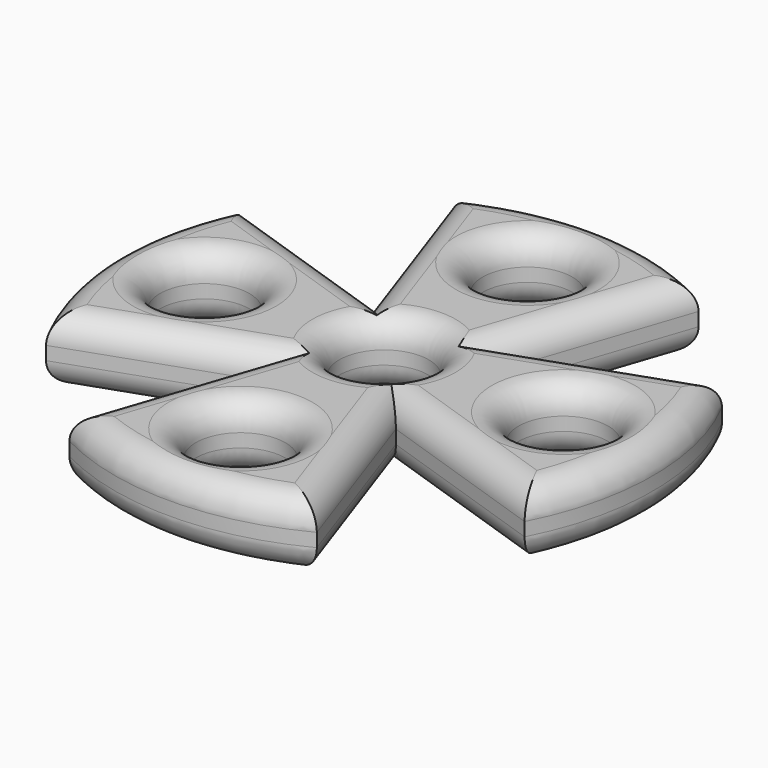
from build123d import *

# Parameters (mm, degrees)
F0_R          = 38.1
F1_DEPTH      = 9.525
F2_R          = 6.35
F3_DEPTH      = 25.4
F4_R          = 6.35
F5_DEPTH      = 25.4
F6_T2_ANGLE   = 83.3157190196
F6_T6_DEPTH   = 45.2852726424
F6_T11_DEPTH  = 45.38242659
F6_T14_ANGLE  = 83.3157190196
F6_T18_DEPTH  = 45.2852726424
F6_T23_DEPTH  = 45.38242659
F6_T26_ANGLE  = 83.3157190196
F6_T30_DEPTH  = 45.2852726424
F6_T35_DEPTH  = 45.38242659
F6_T38_ANGLE  = 83.3157190196
F6_T42_DEPTH  = 45.2852726424
F6_T47_DEPTH  = 45.38242659
F6_T62_DEPTH  = 45.38242659
F6_T65_ANGLE  = 83.3157190196
F6_T69_DEPTH  = 45.2852726424
F6_T74_DEPTH  = 45.38242659
F6_T77_ANGLE  = 83.3157190196
F6_T81_DEPTH  = 45.2852726424
F6_T86_DEPTH  = 45.38242659
F6_T89_ANGLE  = 83.3157190196
F6_T93_DEPTH  = 45.2852726424
F6_T98_DEPTH  = 45.38242659
F6_T101_ANGLE = 83.3157190196
F6_T105_DEPTH = 45.2852726424
F6_T121_DEPTH = 45.2852726424
F6_T125_DEPTH = 45.38242659
F6_T132_DEPTH = 45.2852726424
F6_T136_DEPTH = 45.38242659
F6_T143_DEPTH = 45.2852726424
F6_T147_DEPTH = 45.38242659
F6_T154_DEPTH = 45.2852726424
F6_T158_DEPTH = 45.38242659
F6_T165_DEPTH = 45.2852726424
F6_T169_DEPTH = 45.38242659
F6_T176_DEPTH = 45.2852726424
F6_T180_DEPTH = 45.38242659
F6_T187_DEPTH = 45.2852726424
F6_T191_DEPTH = 45.38242659
F6_T198_DEPTH = 45.2852726424
F6_T202_DEPTH = 45.38242659


# Not quite as in the source:
# - a fillet or chamfer that OpenCascade refuses, or shapes differently, is made with other operations: its cross-section is extruded or revolved along the edge and cut away or added


with BuildPart() as f1:
    # F0 (on Top) → F1 (new body)
    with BuildSketch(Plane.XY):
        Circle(F0_R)
    extrude(amount=F1_DEPTH)

    # F2 (on Top) → F3 (cut)
    with BuildSketch(Plane.XY):
        Circle(F2_R)
    extrude(amount=F3_DEPTH, mode=Mode.SUBTRACT)

    # F4 (on Top) → F5 (cut)
    with BuildSketch(Plane.XY):
        with Locations((-25.4, 0)):
            Circle(F4_R)
        with Locations((0, -25.4)):
            Circle(F4_R)
        with Locations((25.4, 0)):
            Circle(F4_R)
        with Locations((0, 25.4)):
            Circle(F4_R)
        Polygon((-17.7651587874, 34.4617366791), (-44.7468273342, 21.1044754833), (-8.9149055738, 9.045134527), align=None)
        Polygon((-34.4617366791, -17.7651587874), (-21.1044754833, -44.7468273342), (-9.045134527, -8.9149055738), align=None)
        Polygon((17.7651587874, -34.4617366791), (44.7468273342, -21.1044754833), (8.9149055738, -9.045134527), align=None)
        Polygon((34.4617366791, 17.7651587874), (21.1044754833, 44.7468273342), (9.045134527, 8.9149055738), align=None)
    extrude(amount=F5_DEPTH, mode=Mode.SUBTRACT)

    # F6: fillet of radius 3.81 on 34 edges, made by hand

    # F6_s1 → F6_t2 (revolve, cut)
    with BuildSketch(Plane(origin=(0, 0, 0), x_dir=(0, 0, 1), z_dir=(-0.6636019942, -0.7480858195, 0))):
        with BuildLine():
            ThreePointArc((3.81, -38.1), (1.1159231637, -36.9840768363), (0, -34.29))
            Line((0, -34.29), (0, -38.1))
            Line((0, -38.1), (3.81, -38.1))
        make_face()
    revolve(axis=Axis((0, 0, 0), (0, 0, 1)), revolution_arc=F6_T2_ANGLE, mode=Mode.SUBTRACT)


with BuildPart() as f6_tool4:
    # F6_s5 → F6_t6 (new body)
    with BuildSketch(Plane(origin=(1.8403080974, 0.6408092064, 0), x_dir=(0, 0, 1), z_dir=(0.9443849567, 0.3288419887, 0))):
        with BuildLine():
            ThreePointArc((3.81, -5.4446826883), (1.1159231637, -4.3287595247), (0, -1.6346826883))
            Line((0, -1.6346826883), (0, -5.4446826883))
            Line((0, -5.4446826883), (3.81, -5.4446826883))
        make_face()
    extrude(amount=F6_T6_DEPTH)

    split(bisect_by=Plane(origin=(5.4297767191, -1.8274076733, 0), x_dir=(0, 0, 1), z_dir=(0.9477638762, -0.3189727809, 0)), keep=Keep.TOP)


with BuildPart() as f1_1:
    add(f1.part)

    # F6_t3: cut F6_tool4
    add(f6_tool4.part, mode=Mode.SUBTRACT)


with BuildPart() as f6_tool9:
    # F6_s10 → F6_t11 (new body)
    with BuildSketch(Plane(origin=(15.0529008835, 44.7266868627, 0), x_dir=(0, 0, 1), z_dir=(-0.3189727809, -0.9477638762, 0))):
        with BuildLine():
            ThreePointArc((3.81, -5.7290395377), (1.1159231637, -4.613116374), (0, -1.9190395377))
            Line((0, -1.9190395377), (0, -5.7290395377))
            Line((0, -5.7290395377), (3.81, -5.7290395377))
        make_face()
    extrude(amount=F6_T11_DEPTH)

    split(bisect_by=Plane(origin=(-1.7904402831, 5.1418764249, 0), x_dir=(0, 0, 1), z_dir=(-0.3288419887, 0.9443849567, 0)), keep=Keep.TOP)


with BuildPart() as f1_2:
    add(f1_1.part)

    # F6_t8: cut F6_tool9
    add(f6_tool9.part, mode=Mode.SUBTRACT)

    # F6_s13 → F6_t14 (revolve, cut)
    with BuildSketch(Plane(origin=(0, 0, 0), x_dir=(0, 0, 1), z_dir=(0.7480858195, -0.6636019942, 0))):
        with BuildLine():
            ThreePointArc((3.81, -38.1), (1.1159231637, -36.9840768363), (0, -34.29))
            Line((0, -34.29), (0, -38.1))
            Line((0, -38.1), (3.81, -38.1))
        make_face()
    revolve(axis=Axis((0, 0, 0), (0, 0, 1)), revolution_arc=F6_T14_ANGLE, mode=Mode.SUBTRACT)


with BuildPart() as f6_tool16:
    # F6_s17 → F6_t18 (new body)
    with BuildSketch(Plane(origin=(-0.6408092064, 1.8403080974, 0), x_dir=(0, 0, 1), z_dir=(-0.3288419887, 0.9443849567, 0))):
        with BuildLine():
            ThreePointArc((3.81, -5.4446826883), (1.1159231637, -4.3287595247), (0, -1.6346826883))
            Line((0, -1.6346826883), (0, -5.4446826883))
            Line((0, -5.4446826883), (3.81, -5.4446826883))
        make_face()
    extrude(amount=F6_T18_DEPTH)

    split(bisect_by=Plane(origin=(1.8274076733, 5.4297767191, 0), x_dir=(0, 0, 1), z_dir=(0.3189727809, 0.9477638762, 0)), keep=Keep.TOP)


with BuildPart() as f1_3:
    add(f1_2.part)

    # F6_t15: cut F6_tool16
    add(f6_tool16.part, mode=Mode.SUBTRACT)


with BuildPart() as f6_tool21:
    # F6_s22 → F6_t23 (new body)
    with BuildSketch(Plane(origin=(-44.7266868627, 15.0529008835, 0), x_dir=(0, 0, 1), z_dir=(0.9477638762, -0.3189727809, 0))):
        with BuildLine():
            ThreePointArc((3.81, -5.7290395377), (1.1159231637, -4.613116374), (0, -1.9190395377))
            Line((0, -1.9190395377), (0, -5.7290395377))
            Line((0, -5.7290395377), (3.81, -5.7290395377))
        make_face()
    extrude(amount=F6_T23_DEPTH)

    split(bisect_by=Plane(origin=(-5.1418764249, -1.7904402831, 0), x_dir=(0, 0, 1), z_dir=(-0.9443849567, -0.3288419887, 0)), keep=Keep.TOP)


with BuildPart() as f1_4:
    add(f1_3.part)

    # F6_t20: cut F6_tool21
    add(f6_tool21.part, mode=Mode.SUBTRACT)

    # F6_s25 → F6_t26 (revolve, cut)
    with BuildSketch(Plane(origin=(0, 0, 0), x_dir=(0, 0, 1), z_dir=(0.6636019942, 0.7480858195, 0))):
        with BuildLine():
            ThreePointArc((3.81, -38.1), (1.1159231637, -36.9840768363), (0, -34.29))
            Line((0, -34.29), (0, -38.1))
            Line((0, -38.1), (3.81, -38.1))
        make_face()
    revolve(axis=Axis((0, 0, 0), (0, 0, 1)), revolution_arc=F6_T26_ANGLE, mode=Mode.SUBTRACT)


with BuildPart() as f6_tool28:
    # F6_s29 → F6_t30 (new body)
    with BuildSketch(Plane(origin=(-1.8403080974, -0.6408092064, 0), x_dir=(0, 0, 1), z_dir=(-0.9443849567, -0.3288419887, 0))):
        with BuildLine():
            ThreePointArc((3.81, -5.4446826883), (1.1159231637, -4.3287595247), (0, -1.6346826883))
            Line((0, -1.6346826883), (0, -5.4446826883))
            Line((0, -5.4446826883), (3.81, -5.4446826883))
        make_face()
    extrude(amount=F6_T30_DEPTH)

    split(bisect_by=Plane(origin=(-5.4297767191, 1.8274076733, 0), x_dir=(0, 0, 1), z_dir=(-0.9477638762, 0.3189727809, 0)), keep=Keep.TOP)


with BuildPart() as f1_5:
    add(f1_4.part)

    # F6_t27: cut F6_tool28
    add(f6_tool28.part, mode=Mode.SUBTRACT)


with BuildPart() as f6_tool33:
    # F6_s34 → F6_t35 (new body)
    with BuildSketch(Plane(origin=(-15.0529008835, -44.7266868627, 0), x_dir=(0, 0, 1), z_dir=(0.3189727809, 0.9477638762, 0))):
        with BuildLine():
            ThreePointArc((3.81, -5.7290395377), (1.1159231637, -4.613116374), (0, -1.9190395377))
            Line((0, -1.9190395377), (0, -5.7290395377))
            Line((0, -5.7290395377), (3.81, -5.7290395377))
        make_face()
    extrude(amount=F6_T35_DEPTH)

    split(bisect_by=Plane(origin=(1.7904402831, -5.1418764249, 0), x_dir=(0, 0, 1), z_dir=(0.3288419887, -0.9443849567, 0)), keep=Keep.TOP)


with BuildPart() as f1_6:
    add(f1_5.part)

    # F6_t32: cut F6_tool33
    add(f6_tool33.part, mode=Mode.SUBTRACT)

    # F6_s37 → F6_t38 (revolve, cut)
    with BuildSketch(Plane(origin=(0, 0, 0), x_dir=(0, 0, 1), z_dir=(-0.7480858195, 0.6636019942, 0))):
        with BuildLine():
            ThreePointArc((3.81, -38.1), (1.1159231637, -36.9840768363), (0, -34.29))
            Line((0, -34.29), (0, -38.1))
            Line((0, -38.1), (3.81, -38.1))
        make_face()
    revolve(axis=Axis((0, 0, 0), (0, 0, 1)), revolution_arc=F6_T38_ANGLE, mode=Mode.SUBTRACT)


with BuildPart() as f6_tool40:
    # F6_s41 → F6_t42 (new body)
    with BuildSketch(Plane(origin=(0.6408092064, -1.8403080974, 0), x_dir=(0, 0, 1), z_dir=(0.3288419887, -0.9443849567, 0))):
        with BuildLine():
            ThreePointArc((3.81, -5.4446826883), (1.1159231637, -4.3287595247), (0, -1.6346826883))
            Line((0, -1.6346826883), (0, -5.4446826883))
            Line((0, -5.4446826883), (3.81, -5.4446826883))
        make_face()
    extrude(amount=F6_T42_DEPTH)

    split(bisect_by=Plane(origin=(-1.8274076733, -5.4297767191, 0), x_dir=(0, 0, 1), z_dir=(-0.3189727809, -0.9477638762, 0)), keep=Keep.TOP)


with BuildPart() as f1_7:
    add(f1_6.part)

    # F6_t39: cut F6_tool40
    add(f6_tool40.part, mode=Mode.SUBTRACT)


with BuildPart() as f6_tool45:
    # F6_s46 → F6_t47 (new body)
    with BuildSketch(Plane(origin=(44.7266868627, -15.0529008835, 0), x_dir=(0, 0, 1), z_dir=(-0.9477638762, 0.3189727809, 0))):
        with BuildLine():
            ThreePointArc((3.81, -5.7290395377), (1.1159231637, -4.613116374), (0, -1.9190395377))
            Line((0, -1.9190395377), (0, -5.7290395377))
            Line((0, -5.7290395377), (3.81, -5.7290395377))
        make_face()
    extrude(amount=F6_T47_DEPTH)

    split(bisect_by=Plane(origin=(5.1418764249, 1.7904402831, 0), x_dir=(0, 0, 1), z_dir=(0.9443849567, 0.3288419887, 0)), keep=Keep.TOP)


with BuildPart() as f1_8:
    add(f1_7.part)

    # F6_t44: cut F6_tool45
    add(f6_tool45.part, mode=Mode.SUBTRACT)

    # F6_s49 → F6_t50 (revolve, cut)
    with BuildSketch(Plane.XZ.offset(25.4)):
        with BuildLine():
            ThreePointArc((6.35, 3.81), (7.4659231637, 1.1159231637), (10.16, 0))
            Line((10.16, 0), (6.35, 0))
            Line((6.35, 0), (6.35, 3.81))
        make_face()
    revolve(axis=Axis((0, -25.4, 0), (0, 0, 1)), mode=Mode.SUBTRACT)

    # F6_s51 → F6_t52 (revolve, cut)
    with BuildSketch(Plane.XZ):
        with BuildLine():
            ThreePointArc((-19.05, 3.81), (-17.9340768363, 1.1159231637), (-15.24, 0))
            Line((-15.24, 0), (-19.05, 0))
            Line((-19.05, 0), (-19.05, 3.81))
        make_face()
    revolve(axis=Axis((-25.4, 0, 0), (0, 0, 1)), mode=Mode.SUBTRACT)

    # F6_s53 → F6_t54 (revolve, cut)
    with BuildSketch(Plane.XZ):
        with BuildLine():
            ThreePointArc((6.35, 3.81), (7.4659231637, 1.1159231637), (10.16, 0))
            Line((10.16, 0), (6.35, 0))
            Line((6.35, 0), (6.35, 3.81))
        make_face()
    revolve(axis=Axis((0, 0, 0), (0, 0, 1)), mode=Mode.SUBTRACT)

    # F6_s55 → F6_t56 (revolve, cut)
    with BuildSketch(Plane.XZ):
        with BuildLine():
            ThreePointArc((31.75, 3.81), (32.8659231637, 1.1159231637), (35.56, 0))
            Line((35.56, 0), (31.75, 0))
            Line((31.75, 0), (31.75, 3.81))
        make_face()
    revolve(axis=Axis((25.4, 0, 0), (0, 0, 1)), mode=Mode.SUBTRACT)

    # F6_s57 → F6_t58 (revolve, cut)
    with BuildSketch(Plane.XZ.offset(-25.4)):
        with BuildLine():
            ThreePointArc((6.35, 3.81), (7.4659231637, 1.1159231637), (10.16, 0))
            Line((10.16, 0), (6.35, 0))
            Line((6.35, 0), (6.35, 3.81))
        make_face()
    revolve(axis=Axis((0, 25.4, 0), (0, 0, 1)), mode=Mode.SUBTRACT)


with BuildPart() as f6_tool60:
    # F6_s61 → F6_t62 (new body)
    with BuildSketch(Plane(origin=(1.7148623262, -0.5771420697, 0), x_dir=(0, 0, 1), z_dir=(0.9477638762, -0.3189727809, 0))):
        with BuildLine():
            ThreePointArc((9.525, 1.9190395377), (8.4090768363, 4.613116374), (5.715, 5.7290395377))
            Line((5.715, 5.7290395377), (9.525, 5.7290395377))
            Line((9.525, 5.7290395377), (9.525, 1.9190395377))
        make_face()
    extrude(amount=F6_T62_DEPTH)

    split(bisect_by=Plane(origin=(5.1418764249, 1.7904402831, 0), x_dir=(0, 0, 1), z_dir=(0.9443849567, 0.3288419887, 0)), keep=Keep.TOP)


with BuildPart() as f1_9:
    add(f1_8.part)

    # F6_t59: cut F6_tool60
    add(f6_tool60.part, mode=Mode.SUBTRACT)

    # F6_s64 → F6_t65 (revolve, cut)
    with BuildSketch(Plane(origin=(0, 0, 0), x_dir=(0, 0, 1), z_dir=(-0.6657586804, 0.7461671257, 0))):
        with BuildLine():
            ThreePointArc((5.715, 38.1), (8.4090768363, 36.9840768363), (9.525, 34.29))
            Line((9.525, 34.29), (9.525, 38.1))
            Line((9.525, 38.1), (5.715, 38.1))
        make_face()
    revolve(axis=Axis((0, 0, 9.525), (0, 0, -1)), revolution_arc=F6_T65_ANGLE, mode=Mode.SUBTRACT)


with BuildPart() as f6_tool67:
    # F6_s68 → F6_t69 (new body)
    with BuildSketch(Plane(origin=(44.6070383415, 15.5325083215, 0), x_dir=(0, 0, 1), z_dir=(-0.9443849567, -0.3288419887, 0))):
        with BuildLine():
            ThreePointArc((5.715, 5.4446826883), (8.4090768363, 4.3287595247), (9.525, 1.6346826883))
            Line((9.525, 1.6346826883), (9.525, 5.4446826883))
            Line((9.525, 5.4446826883), (5.715, 5.4446826883))
        make_face()
    extrude(amount=F6_T69_DEPTH)

    split(bisect_by=Plane(origin=(5.4297767191, -1.8274076733, 0), x_dir=(0, 0, 1), z_dir=(0.9477638762, -0.3189727809, 0)), keep=Keep.TOP)


with BuildPart() as f1_10:
    add(f1_9.part)

    # F6_t66: cut F6_tool67
    add(f6_tool67.part, mode=Mode.SUBTRACT)


with BuildPart() as f6_tool72:
    # F6_s73 → F6_t74 (new body)
    with BuildSketch(Plane(origin=(0.5771420697, 1.7148623262, 0), x_dir=(0, 0, 1), z_dir=(0.3189727809, 0.9477638762, 0))):
        with BuildLine():
            ThreePointArc((5.715, 5.7290395377), (8.4090768363, 4.613116374), (9.525, 1.9190395377))
            Line((9.525, 1.9190395377), (9.525, 5.7290395377))
            Line((9.525, 5.7290395377), (5.715, 5.7290395377))
        make_face()
    extrude(amount=F6_T74_DEPTH)

    split(bisect_by=Plane(origin=(-1.7904402831, 5.1418764249, 0), x_dir=(0, 0, 1), z_dir=(-0.3288419887, 0.9443849567, 0)), keep=Keep.TOP)


with BuildPart() as f1_11:
    add(f1_10.part)

    # F6_t71: cut F6_tool72
    add(f6_tool72.part, mode=Mode.SUBTRACT)

    # F6_s76 → F6_t77 (revolve, cut)
    with BuildSketch(Plane(origin=(0, 0, 0), x_dir=(0, 0, 1), z_dir=(0.7480858195, -0.6636019942, 0))):
        with BuildLine():
            ThreePointArc((5.715, -38.1), (8.4090768363, -36.9840768363), (9.525, -34.29))
            Line((9.525, -34.29), (9.525, -38.1))
            Line((9.525, -38.1), (5.715, -38.1))
        make_face()
    revolve(axis=Axis((0, 0, 9.525), (0, 0, 1)), revolution_arc=F6_T77_ANGLE, mode=Mode.SUBTRACT)


with BuildPart() as f6_tool79:
    # F6_s80 → F6_t81 (new body)
    with BuildSketch(Plane(origin=(-15.5325083215, 44.6070383415, 0), x_dir=(0, 0, 1), z_dir=(0.3288419887, -0.9443849567, 0))):
        with BuildLine():
            ThreePointArc((5.715, 5.4446826883), (8.4090768363, 4.3287595247), (9.525, 1.6346826883))
            Line((9.525, 1.6346826883), (9.525, 5.4446826883))
            Line((9.525, 5.4446826883), (5.715, 5.4446826883))
        make_face()
    extrude(amount=F6_T81_DEPTH)

    split(bisect_by=Plane(origin=(1.8274076733, 5.4297767191, 0), x_dir=(0, 0, 1), z_dir=(0.3189727809, 0.9477638762, 0)), keep=Keep.TOP)


with BuildPart() as f1_12:
    add(f1_11.part)

    # F6_t78: cut F6_tool79
    add(f6_tool79.part, mode=Mode.SUBTRACT)


with BuildPart() as f6_tool84:
    # F6_s85 → F6_t86 (new body)
    with BuildSketch(Plane(origin=(-1.7148623262, 0.5771420697, 0), x_dir=(0, 0, 1), z_dir=(-0.9477638762, 0.3189727809, 0))):
        with BuildLine():
            ThreePointArc((5.715, 5.7290395377), (8.4090768363, 4.613116374), (9.525, 1.9190395377))
            Line((9.525, 1.9190395377), (9.525, 5.7290395377))
            Line((9.525, 5.7290395377), (5.715, 5.7290395377))
        make_face()
    extrude(amount=F6_T86_DEPTH)

    split(bisect_by=Plane(origin=(-5.1418764249, -1.7904402831, 0), x_dir=(0, 0, 1), z_dir=(-0.9443849567, -0.3288419887, 0)), keep=Keep.TOP)


with BuildPart() as f1_13:
    add(f1_12.part)

    # F6_t83: cut F6_tool84
    add(f6_tool84.part, mode=Mode.SUBTRACT)

    # F6_s88 → F6_t89 (revolve, cut)
    with BuildSketch(Plane(origin=(0, 0, 0), x_dir=(0, 0, 1), z_dir=(0.6636019942, 0.7480858195, 0))):
        with BuildLine():
            ThreePointArc((5.715, -38.1), (8.4090768363, -36.9840768363), (9.525, -34.29))
            Line((9.525, -34.29), (9.525, -38.1))
            Line((9.525, -38.1), (5.715, -38.1))
        make_face()
    revolve(axis=Axis((0, 0, 9.525), (0, 0, 1)), revolution_arc=F6_T89_ANGLE, mode=Mode.SUBTRACT)


with BuildPart() as f6_tool91:
    # F6_s92 → F6_t93 (new body)
    with BuildSketch(Plane(origin=(-44.6070383415, -15.5325083215, 0), x_dir=(0, 0, 1), z_dir=(0.9443849567, 0.3288419887, 0))):
        with BuildLine():
            ThreePointArc((5.715, 5.4446826883), (8.4090768363, 4.3287595247), (9.525, 1.6346826883))
            Line((9.525, 1.6346826883), (9.525, 5.4446826883))
            Line((9.525, 5.4446826883), (5.715, 5.4446826883))
        make_face()
    extrude(amount=F6_T93_DEPTH)

    split(bisect_by=Plane(origin=(-5.4297767191, 1.8274076733, 0), x_dir=(0, 0, 1), z_dir=(-0.9477638762, 0.3189727809, 0)), keep=Keep.TOP)


with BuildPart() as f1_14:
    add(f1_13.part)

    # F6_t90: cut F6_tool91
    add(f6_tool91.part, mode=Mode.SUBTRACT)


with BuildPart() as f6_tool96:
    # F6_s97 → F6_t98 (new body)
    with BuildSketch(Plane(origin=(-0.5771420697, -1.7148623262, 0), x_dir=(0, 0, 1), z_dir=(-0.3189727809, -0.9477638762, 0))):
        with BuildLine():
            ThreePointArc((5.715, 5.7290395377), (8.4090768363, 4.613116374), (9.525, 1.9190395377))
            Line((9.525, 1.9190395377), (9.525, 5.7290395377))
            Line((9.525, 5.7290395377), (5.715, 5.7290395377))
        make_face()
    extrude(amount=F6_T98_DEPTH)

    split(bisect_by=Plane(origin=(1.7904402831, -5.1418764249, 0), x_dir=(0, 0, 1), z_dir=(0.3288419887, -0.9443849567, 0)), keep=Keep.TOP)


with BuildPart() as f1_15:
    add(f1_14.part)

    # F6_t95: cut F6_tool96
    add(f6_tool96.part, mode=Mode.SUBTRACT)

    # F6_s100 → F6_t101 (revolve, cut)
    with BuildSketch(Plane(origin=(0, 0, 0), x_dir=(0, 0, 1), z_dir=(-0.7480858195, 0.6636019942, 0))):
        with BuildLine():
            ThreePointArc((5.715, -38.1), (8.4090768363, -36.9840768363), (9.525, -34.29))
            Line((9.525, -34.29), (9.525, -38.1))
            Line((9.525, -38.1), (5.715, -38.1))
        make_face()
    revolve(axis=Axis((0, 0, 9.525), (0, 0, 1)), revolution_arc=F6_T101_ANGLE, mode=Mode.SUBTRACT)


with BuildPart() as f6_tool103:
    # F6_s104 → F6_t105 (new body)
    with BuildSketch(Plane(origin=(15.5325083215, -44.6070383415, 0), x_dir=(0, 0, 1), z_dir=(-0.3288419887, 0.9443849567, 0))):
        with BuildLine():
            ThreePointArc((5.715, 5.4446826883), (8.4090768363, 4.3287595247), (9.525, 1.6346826883))
            Line((9.525, 1.6346826883), (9.525, 5.4446826883))
            Line((9.525, 5.4446826883), (5.715, 5.4446826883))
        make_face()
    extrude(amount=F6_T105_DEPTH)

    split(bisect_by=Plane(origin=(-1.8274076733, -5.4297767191, 0), x_dir=(0, 0, 1), z_dir=(-0.3189727809, -0.9477638762, 0)), keep=Keep.TOP)


with BuildPart() as f1_16:
    add(f1_15.part)

    # F6_t102: cut F6_tool103
    add(f6_tool103.part, mode=Mode.SUBTRACT)

    # F6_s107 → F6_t108 (revolve, cut)
    with BuildSketch(Plane.XZ.offset(25.4)):
        with BuildLine():
            ThreePointArc((10.16, 9.525), (7.4659231637, 8.4090768363), (6.35, 5.715))
            Line((6.35, 5.715), (6.35, 9.525))
            Line((6.35, 9.525), (10.16, 9.525))
        make_face()
    revolve(axis=Axis((0, -25.4, 9.525), (0, 0, -1)), mode=Mode.SUBTRACT)

    # F6_s109 → F6_t110 (revolve, cut)
    with BuildSketch(Plane.XZ):
        with BuildLine():
            ThreePointArc((-15.24, 9.525), (-17.9340768363, 8.4090768363), (-19.05, 5.715))
            Line((-19.05, 5.715), (-19.05, 9.525))
            Line((-19.05, 9.525), (-15.24, 9.525))
        make_face()
    revolve(axis=Axis((-25.4, 0, 9.525), (0, 0, -1)), mode=Mode.SUBTRACT)

    # F6_s111 → F6_t112 (revolve, cut)
    with BuildSketch(Plane.XZ):
        with BuildLine():
            ThreePointArc((10.16, 9.525), (7.4659231637, 8.4090768363), (6.35, 5.715))
            Line((6.35, 5.715), (6.35, 9.525))
            Line((6.35, 9.525), (10.16, 9.525))
        make_face()
    revolve(axis=Axis((0, 0, 9.525), (0, 0, -1)), mode=Mode.SUBTRACT)

    # F6_s113 → F6_t114 (revolve, cut)
    with BuildSketch(Plane.XZ):
        with BuildLine():
            ThreePointArc((35.56, 9.525), (32.8659231637, 8.4090768363), (31.75, 5.715))
            Line((31.75, 5.715), (31.75, 9.525))
            Line((31.75, 9.525), (35.56, 9.525))
        make_face()
    revolve(axis=Axis((25.4, 0, 9.525), (0, 0, -1)), mode=Mode.SUBTRACT)

    # F6_s115 → F6_t116 (revolve, cut)
    with BuildSketch(Plane.XZ.offset(-25.4)):
        with BuildLine():
            ThreePointArc((10.16, 9.525), (7.4659231637, 8.4090768363), (6.35, 5.715))
            Line((6.35, 5.715), (6.35, 9.525))
            Line((6.35, 9.525), (10.16, 9.525))
        make_face()
    revolve(axis=Axis((0, 25.4, 9.525), (0, 0, -1)), mode=Mode.SUBTRACT)


with BuildPart() as f6_tool119:
    # F6_s120 → F6_t121 (new body)
    with BuildSketch(Plane(origin=(1.8403080974, 0.6408092064, 0), x_dir=(0, 0, 1), z_dir=(0.9443849567, 0.3288419887, 0))):
        with BuildLine():
            ThreePointArc((3.81, -5.4446826883), (1.1159231637, -4.3287595247), (0, -1.6346826883))
            Line((0, -1.6346826883), (0, -5.4446826883))
            Line((0, -5.4446826883), (3.81, -5.4446826883))
        make_face()
    extrude(amount=F6_T121_DEPTH)

    split(bisect_by=Plane(origin=(5.4297767191, -1.8274076733, 0), x_dir=(0, 0, 1), z_dir=(-0.9477638762, 0.3189727809, 0)), keep=Keep.TOP)


with BuildPart() as f6_tool123:
    # F6_s124 → F6_t125 (new body)
    with BuildSketch(Plane(origin=(15.0529008835, 44.7266868627, 0), x_dir=(0, 0, 1), z_dir=(-0.3189727809, -0.9477638762, 0))):
        with BuildLine():
            ThreePointArc((3.81, -5.7290395377), (1.1159231637, -4.613116374), (0, -1.9190395377))
            Line((0, -1.9190395377), (0, -5.7290395377))
            Line((0, -5.7290395377), (3.81, -5.7290395377))
        make_face()
    extrude(amount=F6_T125_DEPTH)

    split(bisect_by=Plane(origin=(-1.7904402831, 5.1418764249, 0), x_dir=(0, 0, 1), z_dir=(0.3288419887, -0.9443849567, 0)), keep=Keep.TOP)


with BuildPart() as f6_tool119_1:
    add(f6_tool119.part)

    # F6_t127: intersect F6_tool123
    add(f6_tool123.part, mode=Mode.INTERSECT)


with BuildPart() as f1_17:
    add(f1_16.part)

    # F6_t117: cut F6_tool119
    add(f6_tool119_1.part, mode=Mode.SUBTRACT)


with BuildPart() as f6_tool130:
    # F6_s131 → F6_t132 (new body)
    with BuildSketch(Plane(origin=(-0.6408092064, 1.8403080974, 0), x_dir=(0, 0, 1), z_dir=(-0.3288419887, 0.9443849567, 0))):
        with BuildLine():
            ThreePointArc((3.81, -5.4446826883), (1.1159231637, -4.3287595247), (0, -1.6346826883))
            Line((0, -1.6346826883), (0, -5.4446826883))
            Line((0, -5.4446826883), (3.81, -5.4446826883))
        make_face()
    extrude(amount=F6_T132_DEPTH)

    split(bisect_by=Plane(origin=(1.8274076733, 5.4297767191, 0), x_dir=(0, 0, 1), z_dir=(-0.3189727809, -0.9477638762, 0)), keep=Keep.TOP)


with BuildPart() as f6_tool134:
    # F6_s135 → F6_t136 (new body)
    with BuildSketch(Plane(origin=(-44.7266868627, 15.0529008835, 0), x_dir=(0, 0, 1), z_dir=(0.9477638762, -0.3189727809, 0))):
        with BuildLine():
            ThreePointArc((3.81, -5.7290395377), (1.1159231637, -4.613116374), (0, -1.9190395377))
            Line((0, -1.9190395377), (0, -5.7290395377))
            Line((0, -5.7290395377), (3.81, -5.7290395377))
        make_face()
    extrude(amount=F6_T136_DEPTH)

    split(bisect_by=Plane(origin=(-5.1418764249, -1.7904402831, 0), x_dir=(0, 0, 1), z_dir=(0.9443849567, 0.3288419887, 0)), keep=Keep.TOP)


with BuildPart() as f6_tool130_1:
    add(f6_tool130.part)

    # F6_t138: intersect F6_tool134
    add(f6_tool134.part, mode=Mode.INTERSECT)


with BuildPart() as f1_18:
    add(f1_17.part)

    # F6_t128: cut F6_tool130
    add(f6_tool130_1.part, mode=Mode.SUBTRACT)


with BuildPart() as f6_tool141:
    # F6_s142 → F6_t143 (new body)
    with BuildSketch(Plane(origin=(-1.8403080974, -0.6408092064, 0), x_dir=(0, 0, 1), z_dir=(-0.9443849567, -0.3288419887, 0))):
        with BuildLine():
            ThreePointArc((3.81, -5.4446826883), (1.1159231637, -4.3287595247), (0, -1.6346826883))
            Line((0, -1.6346826883), (0, -5.4446826883))
            Line((0, -5.4446826883), (3.81, -5.4446826883))
        make_face()
    extrude(amount=F6_T143_DEPTH)

    split(bisect_by=Plane(origin=(-5.4297767191, 1.8274076733, 0), x_dir=(0, 0, 1), z_dir=(0.9477638762, -0.3189727809, 0)), keep=Keep.TOP)


with BuildPart() as f6_tool145:
    # F6_s146 → F6_t147 (new body)
    with BuildSketch(Plane(origin=(-15.0529008835, -44.7266868627, 0), x_dir=(0, 0, 1), z_dir=(0.3189727809, 0.9477638762, 0))):
        with BuildLine():
            ThreePointArc((3.81, -5.7290395377), (1.1159231637, -4.613116374), (0, -1.9190395377))
            Line((0, -1.9190395377), (0, -5.7290395377))
            Line((0, -5.7290395377), (3.81, -5.7290395377))
        make_face()
    extrude(amount=F6_T147_DEPTH)

    split(bisect_by=Plane(origin=(1.7904402831, -5.1418764249, 0), x_dir=(0, 0, 1), z_dir=(-0.3288419887, 0.9443849567, 0)), keep=Keep.TOP)


with BuildPart() as f6_tool141_1:
    add(f6_tool141.part)

    # F6_t149: intersect F6_tool145
    add(f6_tool145.part, mode=Mode.INTERSECT)


with BuildPart() as f1_19:
    add(f1_18.part)

    # F6_t139: cut F6_tool141
    add(f6_tool141_1.part, mode=Mode.SUBTRACT)


with BuildPart() as f6_tool152:
    # F6_s153 → F6_t154 (new body)
    with BuildSketch(Plane(origin=(0.6408092064, -1.8403080974, 0), x_dir=(0, 0, 1), z_dir=(0.3288419887, -0.9443849567, 0))):
        with BuildLine():
            ThreePointArc((3.81, -5.4446826883), (1.1159231637, -4.3287595247), (0, -1.6346826883))
            Line((0, -1.6346826883), (0, -5.4446826883))
            Line((0, -5.4446826883), (3.81, -5.4446826883))
        make_face()
    extrude(amount=F6_T154_DEPTH)

    split(bisect_by=Plane(origin=(-1.8274076733, -5.4297767191, 0), x_dir=(0, 0, 1), z_dir=(0.3189727809, 0.9477638762, 0)), keep=Keep.TOP)


with BuildPart() as f6_tool156:
    # F6_s157 → F6_t158 (new body)
    with BuildSketch(Plane(origin=(44.7266868627, -15.0529008835, 0), x_dir=(0, 0, 1), z_dir=(-0.9477638762, 0.3189727809, 0))):
        with BuildLine():
            ThreePointArc((3.81, -5.7290395377), (1.1159231637, -4.613116374), (0, -1.9190395377))
            Line((0, -1.9190395377), (0, -5.7290395377))
            Line((0, -5.7290395377), (3.81, -5.7290395377))
        make_face()
    extrude(amount=F6_T158_DEPTH)

    split(bisect_by=Plane(origin=(5.1418764249, 1.7904402831, 0), x_dir=(0, 0, 1), z_dir=(-0.9443849567, -0.3288419887, 0)), keep=Keep.TOP)


with BuildPart() as f6_tool152_1:
    add(f6_tool152.part)

    # F6_t160: intersect F6_tool156
    add(f6_tool156.part, mode=Mode.INTERSECT)


with BuildPart() as f1_20:
    add(f1_19.part)

    # F6_t150: cut F6_tool152
    add(f6_tool152_1.part, mode=Mode.SUBTRACT)


with BuildPart() as f6_tool163:
    # F6_s164 → F6_t165 (new body)
    with BuildSketch(Plane(origin=(15.5325083215, -44.6070383415, 0), x_dir=(0, 0, 1), z_dir=(-0.3288419887, 0.9443849567, 0))):
        with BuildLine():
            ThreePointArc((5.715, 5.4446826883), (8.4090768363, 4.3287595247), (9.525, 1.6346826883))
            Line((9.525, 1.6346826883), (9.525, 5.4446826883))
            Line((9.525, 5.4446826883), (5.715, 5.4446826883))
        make_face()
    extrude(amount=F6_T165_DEPTH)

    split(bisect_by=Plane(origin=(-1.8274076733, -5.4297767191, 0), x_dir=(0, 0, 1), z_dir=(0.3189727809, 0.9477638762, 0)), keep=Keep.TOP)


with BuildPart() as f6_tool167:
    # F6_s168 → F6_t169 (new body)
    with BuildSketch(Plane(origin=(1.7148623262, -0.5771420697, 0), x_dir=(0, 0, 1), z_dir=(0.9477638762, -0.3189727809, 0))):
        with BuildLine():
            ThreePointArc((9.525, 1.9190395377), (8.4090768363, 4.613116374), (5.715, 5.7290395377))
            Line((5.715, 5.7290395377), (9.525, 5.7290395377))
            Line((9.525, 5.7290395377), (9.525, 1.9190395377))
        make_face()
    extrude(amount=F6_T169_DEPTH)

    split(bisect_by=Plane(origin=(5.1418764249, 1.7904402831, 0), x_dir=(0, 0, 1), z_dir=(-0.9443849567, -0.3288419887, 0)), keep=Keep.TOP)


with BuildPart() as f6_tool163_1:
    add(f6_tool163.part)

    # F6_t171: intersect F6_tool167
    add(f6_tool167.part, mode=Mode.INTERSECT)


with BuildPart() as f1_21:
    add(f1_20.part)

    # F6_t161: cut F6_tool163
    add(f6_tool163_1.part, mode=Mode.SUBTRACT)


with BuildPart() as f6_tool174:
    # F6_s175 → F6_t176 (new body)
    with BuildSketch(Plane(origin=(44.6070383415, 15.5325083215, 0), x_dir=(0, 0, 1), z_dir=(-0.9443849567, -0.3288419887, 0))):
        with BuildLine():
            ThreePointArc((5.715, 5.4446826883), (8.4090768363, 4.3287595247), (9.525, 1.6346826883))
            Line((9.525, 1.6346826883), (9.525, 5.4446826883))
            Line((9.525, 5.4446826883), (5.715, 5.4446826883))
        make_face()
    extrude(amount=F6_T176_DEPTH)

    split(bisect_by=Plane(origin=(5.4297767191, -1.8274076733, 0), x_dir=(0, 0, 1), z_dir=(-0.9477638762, 0.3189727809, 0)), keep=Keep.TOP)


with BuildPart() as f6_tool178:
    # F6_s179 → F6_t180 (new body)
    with BuildSketch(Plane(origin=(0.5771420697, 1.7148623262, 0), x_dir=(0, 0, 1), z_dir=(0.3189727809, 0.9477638762, 0))):
        with BuildLine():
            ThreePointArc((5.715, 5.7290395377), (8.4090768363, 4.613116374), (9.525, 1.9190395377))
            Line((9.525, 1.9190395377), (9.525, 5.7290395377))
            Line((9.525, 5.7290395377), (5.715, 5.7290395377))
        make_face()
    extrude(amount=F6_T180_DEPTH)

    split(bisect_by=Plane(origin=(-1.7904402831, 5.1418764249, 0), x_dir=(0, 0, 1), z_dir=(0.3288419887, -0.9443849567, 0)), keep=Keep.TOP)


with BuildPart() as f6_tool174_1:
    add(f6_tool174.part)

    # F6_t182: intersect F6_tool178
    add(f6_tool178.part, mode=Mode.INTERSECT)


with BuildPart() as f1_22:
    add(f1_21.part)

    # F6_t172: cut F6_tool174
    add(f6_tool174_1.part, mode=Mode.SUBTRACT)


with BuildPart() as f6_tool185:
    # F6_s186 → F6_t187 (new body)
    with BuildSketch(Plane(origin=(-15.5325083215, 44.6070383415, 0), x_dir=(0, 0, 1), z_dir=(0.3288419887, -0.9443849567, 0))):
        with BuildLine():
            ThreePointArc((5.715, 5.4446826883), (8.4090768363, 4.3287595247), (9.525, 1.6346826883))
            Line((9.525, 1.6346826883), (9.525, 5.4446826883))
            Line((9.525, 5.4446826883), (5.715, 5.4446826883))
        make_face()
    extrude(amount=F6_T187_DEPTH)

    split(bisect_by=Plane(origin=(1.8274076733, 5.4297767191, 0), x_dir=(0, 0, 1), z_dir=(-0.3189727809, -0.9477638762, 0)), keep=Keep.TOP)


with BuildPart() as f6_tool189:
    # F6_s190 → F6_t191 (new body)
    with BuildSketch(Plane(origin=(-1.7148623262, 0.5771420697, 0), x_dir=(0, 0, 1), z_dir=(-0.9477638762, 0.3189727809, 0))):
        with BuildLine():
            ThreePointArc((5.715, 5.7290395377), (8.4090768363, 4.613116374), (9.525, 1.9190395377))
            Line((9.525, 1.9190395377), (9.525, 5.7290395377))
            Line((9.525, 5.7290395377), (5.715, 5.7290395377))
        make_face()
    extrude(amount=F6_T191_DEPTH)

    split(bisect_by=Plane(origin=(-5.1418764249, -1.7904402831, 0), x_dir=(0, 0, 1), z_dir=(0.9443849567, 0.3288419887, 0)), keep=Keep.TOP)


with BuildPart() as f6_tool185_1:
    add(f6_tool185.part)

    # F6_t193: intersect F6_tool189
    add(f6_tool189.part, mode=Mode.INTERSECT)


with BuildPart() as f1_23:
    add(f1_22.part)

    # F6_t183: cut F6_tool185
    add(f6_tool185_1.part, mode=Mode.SUBTRACT)


with BuildPart() as f6_tool196:
    # F6_s197 → F6_t198 (new body)
    with BuildSketch(Plane(origin=(-44.6070383415, -15.5325083215, 0), x_dir=(0, 0, 1), z_dir=(0.9443849567, 0.3288419887, 0))):
        with BuildLine():
            ThreePointArc((5.715, 5.4446826883), (8.4090768363, 4.3287595247), (9.525, 1.6346826883))
            Line((9.525, 1.6346826883), (9.525, 5.4446826883))
            Line((9.525, 5.4446826883), (5.715, 5.4446826883))
        make_face()
    extrude(amount=F6_T198_DEPTH)

    split(bisect_by=Plane(origin=(-5.4297767191, 1.8274076733, 0), x_dir=(0, 0, 1), z_dir=(0.9477638762, -0.3189727809, 0)), keep=Keep.TOP)


with BuildPart() as f6_tool200:
    # F6_s201 → F6_t202 (new body)
    with BuildSketch(Plane(origin=(-0.5771420697, -1.7148623262, 0), x_dir=(0, 0, 1), z_dir=(-0.3189727809, -0.9477638762, 0))):
        with BuildLine():
            ThreePointArc((5.715, 5.7290395377), (8.4090768363, 4.613116374), (9.525, 1.9190395377))
            Line((9.525, 1.9190395377), (9.525, 5.7290395377))
            Line((9.525, 5.7290395377), (5.715, 5.7290395377))
        make_face()
    extrude(amount=F6_T202_DEPTH)

    split(bisect_by=Plane(origin=(1.7904402831, -5.1418764249, 0), x_dir=(0, 0, 1), z_dir=(-0.3288419887, 0.9443849567, 0)), keep=Keep.TOP)


with BuildPart() as f6_tool196_1:
    add(f6_tool196.part)

    # F6_t204: intersect F6_tool200
    add(f6_tool200.part, mode=Mode.INTERSECT)


with BuildPart() as f1_24:
    add(f1_23.part)

    # F6_t194: cut F6_tool196
    add(f6_tool196_1.part, mode=Mode.SUBTRACT)


solid = f1_24.part
